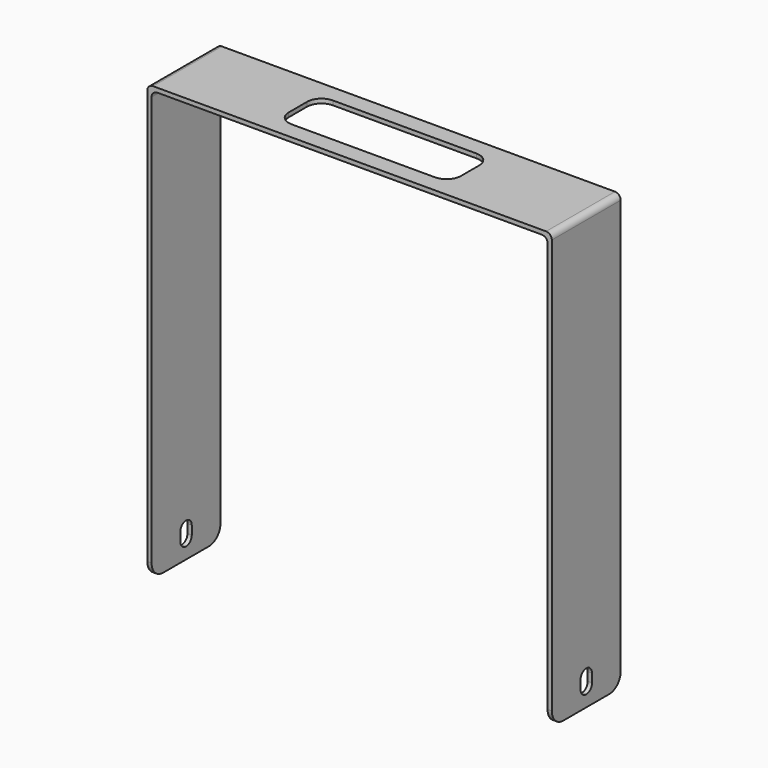
from build123d import *

# Parameters (mm, degrees)
F0_W     = 141
F0_H     = 30
F0_W_2   = 60
F0_H_2   = 18
F1_DEPTH = 1.5
F2_W     = 1.5
F2_H     = 30
F3_DEPTH = 150
F4_R     = 5
F7_DEPTH = 200
F8_R     = 2


# Not quite as in the source:
# - two fillets or chamfers of one size are made in one step


with BuildPart() as f1:
    # F0 (on Top) → F1 (new body)
    with BuildSketch(Plane.XY):
        Rectangle(F0_W, F0_H)
        Rectangle(F0_W_2, F0_H_2, mode=Mode.SUBTRACT)
    extrude(amount=F1_DEPTH)

    # F2 (on face) → F3 (join)
    with BuildSketch(Plane(origin=(0, 0, 0), x_dir=(1, 0, 0), z_dir=(0, 0, -1))):
        with Locations((-69.75, 0)):
            Rectangle(F2_W, F2_H)
        with Locations((69.75, 0)):
            Rectangle(F2_W, F2_H)
    extrude(amount=F3_DEPTH)

    # F4
    f4_edges = [f1.edges().sort_by_distance(p)[0] for p in [
        (30, 9, 0.75),
        (30, -9, 0.75),
        (-30, -9, 0.75),
        (-30, 9, 0.75),
        (-69.75, 15, -150),
        (69.75, 15, -150),
        (69.75, -15, -150),
        (-69.75, -15, -150),
    ]]
    fillet(f4_edges, radius=F4_R)

    # F6 (on face) → F7 (cut)
    with BuildSketch(Plane(origin=(-70.5, 0, 0), x_dir=(0, -1, 0), z_dir=(-1, 0, 0))):
        with BuildLine():
            Line((-2.5, -140.5), (-2.5, -143.5))
            ThreePointArc((-2.5, -143.5), (-1.767766953, -145.267766953), (0, -146))
            ThreePointArc((0, -146), (1.767766953, -145.267766953), (2.5, -143.5))
            Line((2.5, -143.5), (2.5, -140.5))
            ThreePointArc((2.5, -140.5), (1.767766953, -138.732233047), (0, -138))
            ThreePointArc((0, -138), (-1.767766953, -138.732233047), (-2.5, -140.5))
        make_face()
    extrude(amount=-F7_DEPTH, mode=Mode.SUBTRACT)

    # F8
    f8_edges = [f1.edges().sort_by_distance(p)[0] for p in [
        (70.5, 0, 1.5),
        (-70.5, 0, 1.5),
        (-69, 0, 0),
        (69, 0, 0),
    ]]
    fillet(f8_edges, radius=F8_R)


solid = f1.part
